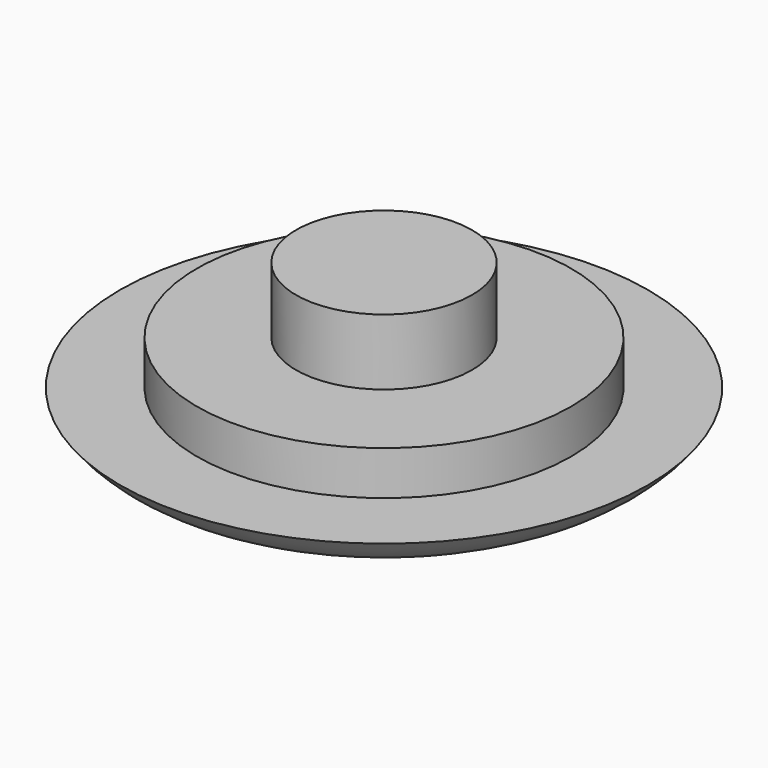
from build123d import *

# Parameters (mm, degrees)
F0_R     = 12
F0_R_2   = 8.5
F1_DEPTH = 2
F0_R_3   = 4
F2_DEPTH = 4
F3_DEPTH = 7


# Not quite as in the source:
# - a fillet or chamfer that OpenCascade refuses, or shapes differently, is made with other operations: its cross-section is extruded or revolved along the edge and cut away or added


with BuildPart() as f1:
    # F0 (on Top) → F1 (new body)
    with BuildSketch(Plane.XY):
        Circle(F0_R)
        Circle(F0_R_2, mode=Mode.SUBTRACT)
    extrude(amount=F1_DEPTH)

    # F0 (on Top) → F2 (join)
    with BuildSketch(Plane.XY):
        Circle(F0_R_2)
        Circle(F0_R_3, mode=Mode.SUBTRACT)
    extrude(amount=F2_DEPTH)

    # F0 (on Top) → F3 (join)
    with BuildSketch(Plane.XY):
        Circle(F0_R_3)
    extrude(amount=F3_DEPTH)

    # F4: fillet of radius 5 on 1 edges, made by hand

    # F4_s1 → F4_t2 (revolve, cut)
    with BuildSketch(Plane.XZ):
        with BuildLine():
            ThreePointArc((12, 2), (10.2360679775, 0.527864045), (8, 0))
            Line((8, 0), (12, 0))
            Line((12, 0), (12, 2))
        make_face()
    revolve(axis=Axis((0, 0, 0), (0, 0, 1)), mode=Mode.SUBTRACT)


solid = f1.part
